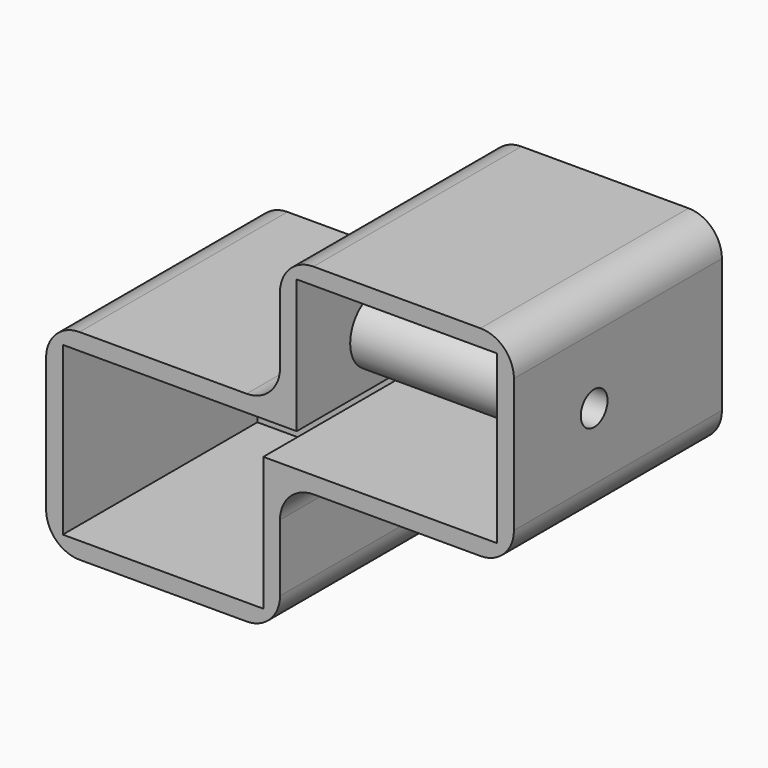
from build123d import *

# Parameters (mm, degrees)
F1_DEPTH    = 38.9
F3_D        = 5
F4_T        = -2.5
F5_T1_DEPTH = 38.9
F5_T6_DEPTH = 38.9
F5_S7_R     = 2.5
F5_T8_DEPTH = 21
F5_T9_DEPTH = 63.9


# Not quite as in the source:
# - a fillet or chamfer that OpenCascade refuses, or shapes differently, is made with other operations: its cross-section is extruded or revolved along the edge and cut away or added


with BuildPart() as f1:
    # F0 (on Front) → F1 (new body)
    with BuildSketch(Plane.XZ):
        Polygon((0, 10), (0, 0), (35, 0), (35, 30), (0, 30), align=None)
        Polygon((0, -20), (0, 0), (0, 10), (-35, 10), (-35, -20), align=None)
    extrude(amount=-F1_DEPTH)

    # F3 (through all)
    with Locations(Plane.YZ.offset(35)):
        with Locations((15, 15)):
            Hole(F3_D / 2)

    # F4
    f4_openings = [f1.faces().sort_by_distance(p)[0] for p in [
        (0, 0, 5),
    ]]
    offset(amount=F4_T, openings=f4_openings, kind=Kind.INTERSECTION)

    # F5: fillet of radius 5 on 8 edges, made by hand

    # F5_s2 → F5_t1 (join)
    with BuildSketch(Plane.XZ.offset(-38.9)):
        with BuildLine():
            ThreePointArc((5, 0), (1.4644660941, -1.4644660941), (0, -5))
            Line((0, -5), (0, 0))
            Line((0, 0), (5, 0))
        make_face()
    extrude(amount=F5_T1_DEPTH)


with BuildPart() as f5_tool4:
    # F5_s5 → F5_t6 (new body)
    with BuildSketch(Plane.XZ):
        with BuildLine():
            ThreePointArc((0, 15), (-1.4644660941, 11.4644660941), (-5, 10))
            Line((-5, 10), (0, 10))
            Line((0, 10), (0, 15))
        make_face()
    extrude(amount=-F5_T6_DEPTH)

    # F5_s7 → F5_t8 (cut, symmetric)
    with BuildSketch(Plane.YZ.offset(-2.5)):
        with Locations((15, 15)):
            Circle(F5_S7_R)
    extrude(amount=F5_T8_DEPTH, both=True, mode=Mode.SUBTRACT)


with BuildPart() as f1_1:
    add(f1.part)

    # F5_t3: union F5_tool4
    add(f5_tool4.part)

    # F5_s10 → F5_t9 (cut)
    with BuildSketch(Plane.XZ.offset(-51.4)):
        with BuildLine():
            ThreePointArc((-30, 10), (-33.5355339059, 8.5355339059), (-35, 5))
            Line((-35, 5), (-35, 10))
            Line((-35, 10), (-30, 10))
        make_face()
        with BuildLine():
            ThreePointArc((-5, -20), (-1.4644660941, -18.5355339059), (0, -15))
            Line((0, -15), (0, -20))
            Line((0, -20), (-5, -20))
        make_face()
        with BuildLine():
            ThreePointArc((30, 0), (33.5355339059, 1.4644660941), (35, 5))
            Line((35, 5), (35, 0))
            Line((35, 0), (30, 0))
        make_face()
        with BuildLine():
            ThreePointArc((5, 30), (1.4644660941, 28.5355339059), (0, 25))
            Line((0, 25), (0, 30))
            Line((0, 30), (5, 30))
        make_face()
        with BuildLine():
            ThreePointArc((-35, -15), (-33.5355339059, -18.5355339059), (-30, -20))
            Line((-30, -20), (-35, -20))
            Line((-35, -20), (-35, -15))
        make_face()
        with BuildLine():
            ThreePointArc((35, 25), (33.5355339059, 28.5355339059), (30, 30))
            Line((30, 30), (35, 30))
            Line((35, 30), (35, 25))
        make_face()
    extrude(amount=F5_T9_DEPTH, mode=Mode.SUBTRACT)


solid = f1_1.part
